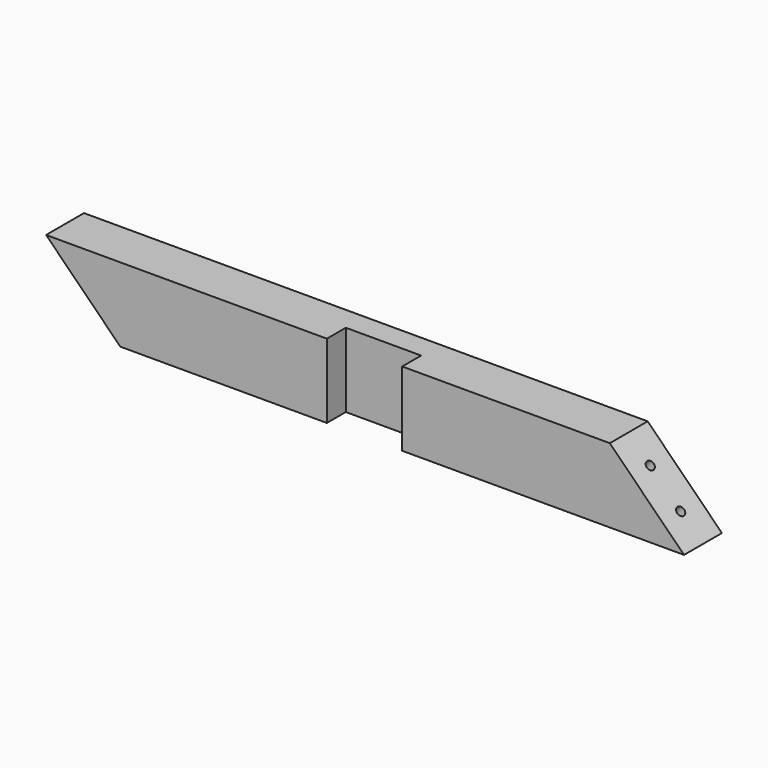
from build123d import *

# Parameters (mm, degrees)
F0_W     = 44
F0_H     = 69
F1_DEPTH = 593
F2_SIZE  = 68.99999
F4_D     = 8
F4_DEPTH = 20
F4_TIP   = 2.4034424761
F5_SIZE  = 68.99999
F7_D     = 8
F7_DEPTH = 20
F7_TIP   = 2.4034424761
F8_W     = 70
F8_H     = 69
F9_DEPTH = 22


# Not quite as in the source:
# - a fillet or chamfer is up to 0.001 mm smaller than in the source, because OpenCascade refuses the exact size


with BuildPart() as f1:
    # F0 (on Right) → F1 (new body)
    with BuildSketch(Plane.YZ):
        with Locations((2.3388881236, 4.4023249735)):
            Rectangle(F0_W, F0_H)
    extrude(amount=F1_DEPTH)

    # F2 (size 69 in the source; OpenCascade refuses exactly that, so slightly less here)
    f2_edges = [f1.edges().sort_by_distance(p)[0] for p in [
        (0, 2.338888, -30.097675),
    ]]
    chamfer(f2_edges, length=F2_SIZE)

    # F4
    with Locations(Plane(origin=(19.4511624867, 0, 19.4511624867), x_dir=(0, -1, 0), z_dir=(-0.7071067812, 0, -0.7071067812))):
        with Locations((-2.3388881236, 0), (-2.3388881236, -40)):
            Hole(F4_D / 2, depth=F4_DEPTH)
            with Locations((0, 0, -(F4_DEPTH + F4_TIP / 2))):  # 118° drill point
                Cone(0, F4_D / 2, F4_TIP, mode=Mode.SUBTRACT)

    # F5 (size 69 in the source; OpenCascade refuses exactly that, so slightly less here)
    f5_edges = [f1.edges().sort_by_distance(p)[0] for p in [
        (593, 2.338888, 38.902325),
    ]]
    chamfer(f5_edges, length=F5_SIZE)

    # F7
    with Locations(Plane(origin=(281.4511624867, 0, 281.4511624867), x_dir=(0, 1, 0), z_dir=(0.7071067812, 0, 0.7071067812))):
        with Locations((1.8450106473, -371.8575412992), (1.8450106473, -411.8575412992)):
            Hole(F7_D / 2, depth=F7_DEPTH)
            with Locations((0, 0, -(F7_DEPTH + F7_TIP / 2))):  # 118° drill point
                Cone(0, F7_D / 2, F7_TIP, mode=Mode.SUBTRACT)

    # F8 (on face) → F9 (cut)
    with BuildSketch(Plane.XZ.offset(19.6611118764)):
        with Locations((296, 4.4023249735)):
            Rectangle(F8_W, F8_H)
    extrude(amount=-F9_DEPTH, mode=Mode.SUBTRACT)


solid = f1.part
